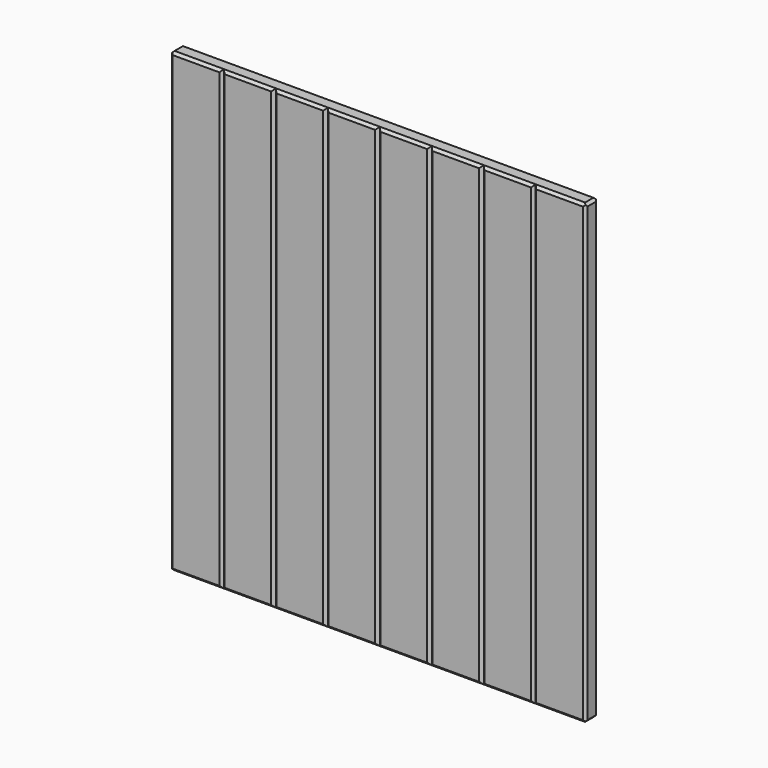
from build123d import *

# Parameters (mm, degrees)
F0_W      = 508
F0_H      = 558.8
F1_DEPTH  = 19.05
F3_DEPTH  = 558.801
F4_SIZE   = 3.17499
F5_SIZE   = 3.175
F7_DEPTH  = 558.801
F8_SIZE   = 3.17499
F8_SIZE_2 = 3.175


# Not quite as in the source:
# - a fillet or chamfer is up to 0.001 mm smaller than in the source, because OpenCascade refuses the exact size


with BuildPart() as f1:
    # F0 (on Front) → F1 (new body)
    with BuildSketch(Plane.XZ):
        Rectangle(F0_W, F0_H)
    extrude(amount=F1_DEPTH)

    # F2 (on face) → F3 (cut, through all)
    with BuildSketch(Plane(origin=(0, 0, -279.4), x_dir=(1, 0, 0), z_dir=(0, 0, -1))):
        Polygon((190.5, 19.05), (187.325, 19.05), (190.5, 15.875), (193.675, 19.05), align=None)
        Polygon((127, 19.05), (123.825, 19.05), (127, 15.875), (130.175, 19.05), align=None)
        Polygon((63.5, 19.05), (60.325, 19.05), (63.5, 15.875), (66.675, 19.05), align=None)
        Polygon((0, 19.05), (-3.175, 19.05), (0, 15.875), (3.175, 19.05), align=None)
        Polygon((-63.5, 19.05), (-66.675, 19.05), (-63.5, 15.875), (-60.325, 19.05), align=None)
        Polygon((-127, 19.05), (-130.175, 19.05), (-127, 15.875), (-123.825, 19.05), align=None)
        Polygon((-190.5, 19.05), (-193.675, 19.05), (-190.5, 15.875), (-187.325, 19.05), align=None)
    extrude(amount=-F3_DEPTH, mode=Mode.SUBTRACT)

    # F4 (size 3.175 in the source; OpenCascade refuses exactly that, so slightly less here)
    f4_edges = [f1.edges().sort_by_distance(p)[0] for p in [
        (-254, -19.05, 0),
        (-223.8375, -19.05, -279.4),
        (-158.75, -19.05, -279.4),
        (-95.25, -19.05, -279.4),
        (-31.75, -19.05, -279.4),
        (31.75, -19.05, -279.4),
        (95.25, -19.05, -279.4),
        (158.75, -19.05, -279.4),
        (223.8375, -19.05, -279.4),
        (254, -19.05, 0),
        (223.8375, -19.05, 279.4),
        (158.75, -19.05, 279.4),
        (95.25, -19.05, 279.4),
        (31.75, -19.05, 279.4),
        (-31.75, -19.05, 279.4),
        (-95.25, -19.05, 279.4),
        (-158.75, -19.05, 279.4),
        (-223.8375, -19.05, 279.4),
    ]]
    chamfer(f4_edges, length=F4_SIZE)

    # F5
    f5_edges = [f1.edges().sort_by_distance(p)[0] for p in [
        (-254, -7.937505, 279.4),
        (-254, -7.937505, -279.4),
        (254, -7.937505, -279.4),
        (254, -7.937505, 279.4),
    ]]
    chamfer(f5_edges, length=F5_SIZE)

    # F6 (on face) → F7 (cut, through all)
    with BuildSketch(Plane(origin=(0, 0, -279.4), x_dir=(1, 0, 0), z_dir=(0, 0, -1))):
        Polygon((-193.675, 0), (-190.5, 0), (-187.325, 0), (-190.5, 3.175), align=None)
        Polygon((-123.825, 0), (-127, 3.175), (-130.175, 0), (-127, 0), align=None)
        Polygon((-60.325, 0), (-63.5, 3.175), (-66.675, 0), (-63.5, 0), align=None)
        Polygon((3.175, 0), (0, 3.175), (-3.175, 0), (0, 0), align=None)
        Polygon((66.675, 0), (63.5, 3.175), (60.325, 0), (63.5, 0), align=None)
        Polygon((130.175, 0), (127, 3.175), (123.825, 0), (127, 0), align=None)
        Polygon((193.675, 0), (190.5, 3.175), (187.325, 0), (190.5, 0), align=None)
    extrude(amount=-F7_DEPTH, mode=Mode.SUBTRACT)

    # F8 (call 1 of 18: OpenCascade refuses the feature's edges together) (size 3.175 in the source; OpenCascade refuses exactly that, so slightly less here)
    f8_edges = [f1.edges().sort_by_distance(p)[0] for p in [
        (-222.25, 0, -279.4),
    ]]
    chamfer(f8_edges, length=F8_SIZE)

    # F8#2 (call 2 of 18)
    f8_2_edges = [f1.edges().sort_by_distance(p)[0] for p in [
        (-254, 0, 0),
    ]]
    chamfer(f8_2_edges, length=F8_SIZE_2)

    # F8#3 (call 3 of 18) (size 3.175 in the source; OpenCascade refuses exactly that, so slightly less here)
    f8_3_edges = [f1.edges().sort_by_distance(p)[0] for p in [
        (-158.75, 0, -279.4),
    ]]
    chamfer(f8_3_edges, length=F8_SIZE)

    # F8#4 (call 4 of 18) (size 3.175 in the source; OpenCascade refuses exactly that, so slightly less here)
    f8_4_edges = [f1.edges().sort_by_distance(p)[0] for p in [
        (-95.25, 0, -279.4),
    ]]
    chamfer(f8_4_edges, length=F8_SIZE)

    # F8#5 (call 5 of 18) (size 3.175 in the source; OpenCascade refuses exactly that, so slightly less here)
    f8_5_edges = [f1.edges().sort_by_distance(p)[0] for p in [
        (-31.75, 0, -279.4),
    ]]
    chamfer(f8_5_edges, length=F8_SIZE)

    # F8#6 (call 6 of 18) (size 3.175 in the source; OpenCascade refuses exactly that, so slightly less here)
    f8_6_edges = [f1.edges().sort_by_distance(p)[0] for p in [
        (31.75, 0, -279.4),
    ]]
    chamfer(f8_6_edges, length=F8_SIZE)

    # F8#7 (call 7 of 18) (size 3.175 in the source; OpenCascade refuses exactly that, so slightly less here)
    f8_7_edges = [f1.edges().sort_by_distance(p)[0] for p in [
        (95.25, 0, -279.4),
    ]]
    chamfer(f8_7_edges, length=F8_SIZE)

    # F8#8 (call 8 of 18) (size 3.175 in the source; OpenCascade refuses exactly that, so slightly less here)
    f8_8_edges = [f1.edges().sort_by_distance(p)[0] for p in [
        (158.75, 0, -279.4),
    ]]
    chamfer(f8_8_edges, length=F8_SIZE)

    # F8#9 (call 9 of 18) (size 3.175 in the source; OpenCascade refuses exactly that, so slightly less here)
    f8_9_edges = [f1.edges().sort_by_distance(p)[0] for p in [
        (222.25, 0, -279.4),
    ]]
    chamfer(f8_9_edges, length=F8_SIZE)

    # F8#10 (call 10 of 18)
    f8_10_edges = [f1.edges().sort_by_distance(p)[0] for p in [
        (254, 0, 0),
    ]]
    chamfer(f8_10_edges, length=F8_SIZE_2)

    # F8#11 (call 11 of 18) (size 3.175 in the source; OpenCascade refuses exactly that, so slightly less here)
    f8_11_edges = [f1.edges().sort_by_distance(p)[0] for p in [
        (222.25, 0, 279.4),
    ]]
    chamfer(f8_11_edges, length=F8_SIZE)

    # F8#12 (call 12 of 18) (size 3.175 in the source; OpenCascade refuses exactly that, so slightly less here)
    f8_12_edges = [f1.edges().sort_by_distance(p)[0] for p in [
        (158.75, 0, 279.4),
    ]]
    chamfer(f8_12_edges, length=F8_SIZE)

    # F8#13 (call 13 of 18) (size 3.175 in the source; OpenCascade refuses exactly that, so slightly less here)
    f8_13_edges = [f1.edges().sort_by_distance(p)[0] for p in [
        (95.25, 0, 279.4),
    ]]
    chamfer(f8_13_edges, length=F8_SIZE)

    # F8#14 (call 14 of 18) (size 3.175 in the source; OpenCascade refuses exactly that, so slightly less here)
    f8_14_edges = [f1.edges().sort_by_distance(p)[0] for p in [
        (31.75, 0, 279.4),
    ]]
    chamfer(f8_14_edges, length=F8_SIZE)

    # F8#15 (call 15 of 18) (size 3.175 in the source; OpenCascade refuses exactly that, so slightly less here)
    f8_15_edges = [f1.edges().sort_by_distance(p)[0] for p in [
        (-31.75, 0, 279.4),
    ]]
    chamfer(f8_15_edges, length=F8_SIZE)

    # F8#16 (call 16 of 18) (size 3.175 in the source; OpenCascade refuses exactly that, so slightly less here)
    f8_16_edges = [f1.edges().sort_by_distance(p)[0] for p in [
        (-95.25, 0, 279.4),
    ]]
    chamfer(f8_16_edges, length=F8_SIZE)

    # F8#17 (call 17 of 18) (size 3.175 in the source; OpenCascade refuses exactly that, so slightly less here)
    f8_17_edges = [f1.edges().sort_by_distance(p)[0] for p in [
        (-158.75, 0, 279.4),
    ]]
    chamfer(f8_17_edges, length=F8_SIZE)

    # F8#18 (call 18 of 18) (size 3.175 in the source; OpenCascade refuses exactly that, so slightly less here)
    f8_18_edges = [f1.edges().sort_by_distance(p)[0] for p in [
        (-222.25, 0, 279.4),
    ]]
    chamfer(f8_18_edges, length=F8_SIZE)


solid = f1.part
